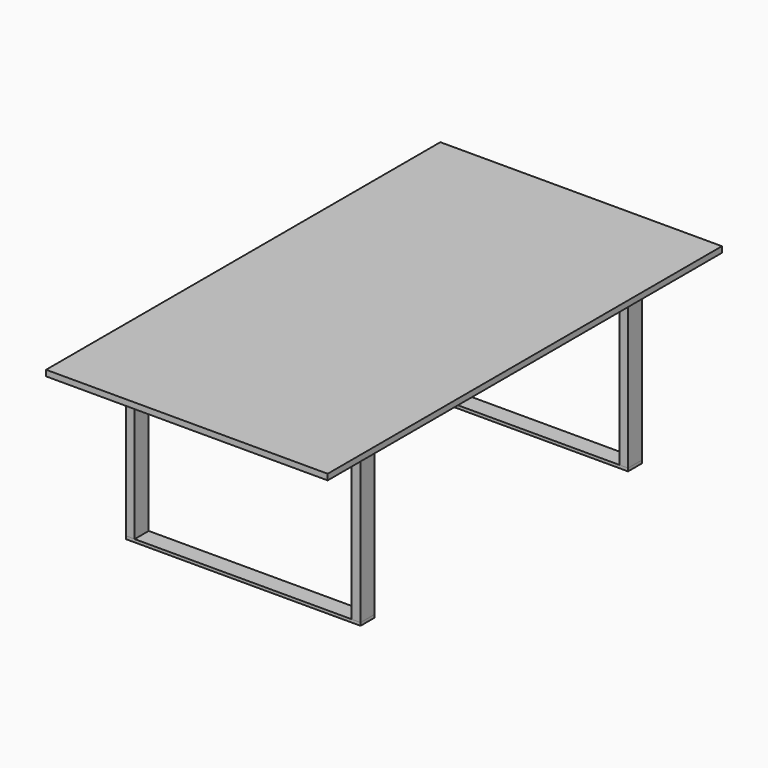
from build123d import *

# Parameters (mm, degrees)
F0_W      = 1219.2
F0_H      = 2133.6
F1_DEPTH  = 25.4
F2_W      = 25.4
F2_H      = 1524
F3_DEPTH  = 50.8
F5_W      = 1016
F5_H      = 25.4
F6_DEPTH  = 50.8
F8_W      = 76.2
F8_H      = 711.2
F9_DEPTH  = 38.1
F12_W     = 1016
F12_H     = 76.2
F13_DEPTH = 12.7
F15_W     = 25.4
F15_H     = 1524
F16_DEPTH = 50.8


# Not quite as in the source:
# - a feature names something its author has since deleted; it is built from what else it names


with BuildPart() as f1:
    # F0 (on Top) → F1 (new body)
    with BuildSketch(Plane.XY):
        Rectangle(F0_W, F0_H)
    extrude(amount=F1_DEPTH)


with BuildPart() as f3:
    # F2 (on face) → F3 (new body)
    with BuildSketch(Plane.XY):
        with Locations((495.3, 0)):
            Rectangle(F2_W, F2_H)
    extrude(amount=-F3_DEPTH)


with BuildPart() as f4_1:
    # F4: instance of F3
    add(f3.part.mirror(Plane.YZ))


with BuildPart() as f6:
    # F5 (on face) → F6 (new body)
    with BuildSketch(Plane.XY):
        with Locations((0, -749.3)):
            Rectangle(F5_W, F5_H)
    extrude(amount=-F6_DEPTH)


with BuildPart() as f7_1:
    # F7: instance of F6
    add(f6.part.mirror(Plane.XZ))


with BuildPart() as f9:
    # F8 (on face) → F9 (new body)
    with BuildSketch(Plane(origin=(-508, 0, 0), x_dir=(0, -1, 0), z_dir=(-1, 0, 0))):
        with Locations((-723.9, -355.6)):
            Rectangle(F8_W, F8_H)
    extrude(amount=-F9_DEPTH)


with BuildPart() as f10_1:
    # F10: instance of F9
    add(f9.part.mirror(Plane.YZ))


with BuildPart() as f11_1:
    # F11: instance of F10_1
    add(f10_1.part.mirror(Plane.XZ))


with BuildPart() as f11_2:
    # F11: instance of F9
    add(f9.part.mirror(Plane.XZ))


with BuildPart() as f13:
    # F12 (on face) → F13 (new body)
    with BuildSketch(Plane(origin=(0, 0, -711.2), x_dir=(1, 0, 0), z_dir=(0, 0, -1))):
        with Locations((0, 723.9)):
            Rectangle(F12_W, F12_H)
    extrude(amount=-F13_DEPTH)


with BuildPart() as f14_1:
    # F14: instance of F13
    add(f13.part.mirror(Plane.XZ))


with BuildPart() as f16:
    # F15 (on face) → F16 (new body)
    with BuildSketch(Plane.XY):
        with Locations((-190.5, 0)):
            Rectangle(F15_W, F15_H)
    extrude(amount=-F16_DEPTH)


with BuildPart() as f17_1:
    # F17: instance of F16
    add(f16.part.mirror(Plane.YZ))


solid = Compound([f1.part, f3.part, f4_1.part, f6.part, f7_1.part, f9.part, f10_1.part, f11_1.part, f11_2.part, f13.part, f14_1.part, f16.part, f17_1.part])
